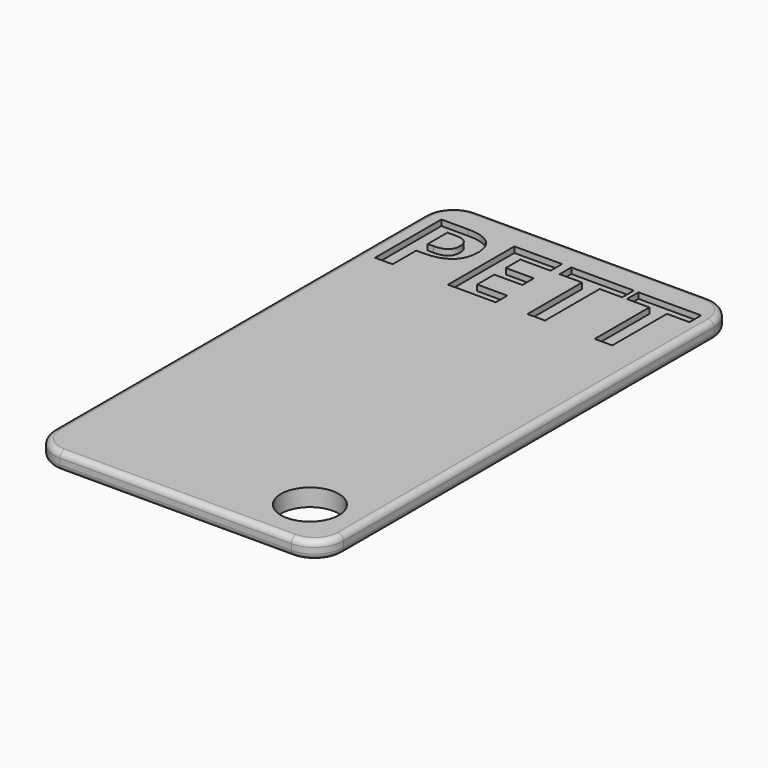
from build123d import *

# Parameters (mm, degrees)
F0_W         = 90
F0_H         = 50
F1_DEPTH     = 3
F2_R         = 1
F3_T1_DEPTH  = 3
F3_T4_ANGLE  = 90
F3_T6_ANGLE  = 90
F3_T8_ANGLE  = 90
F3_T10_ANGLE = 90
F3_T12_ANGLE = 90
F3_T14_ANGLE = 90
F3_T16_ANGLE = 90
F3_T18_ANGLE = 90
F5_ANGLE     = 90
F6_TEXT_SIZE = 20.075807084
F7_DEPTH     = 1
F8_R         = 5
F9_DEPTH     = 3


# Not quite as in the source:
# - a fillet or chamfer that OpenCascade refuses, or shapes differently, is made with other operations: its cross-section is extruded or revolved along the edge and cut away or added
# - Text() gives the source's letters only with a copy of the font that has no kerning and outlines rounded to 1/6400 em; it was checked with that copy


with BuildPart() as f1:
    # F0 (on Top) → F1 (new body)
    with BuildSketch(Plane.XY):
        Rectangle(F0_W, F0_H)
    extrude(amount=F1_DEPTH)

    # F2
    f2_edges = [f1.edges().sort_by_distance(p)[0] for p in [
        (0, 25, 3),
        (-45, 0, 3),
        (0, -25, 3),
        (45, 0, 3),
        (0, 25, 0),
        (-45, 0, 0),
        (0, -25, 0),
        (45, 0, 0),
    ]]
    fillet(f2_edges, radius=F2_R)

    # F3: fillet of radius 5 on 4 edges, made by hand

    # F3_s2 → F3_t1 (cut)
    with BuildSketch(Plane.XY):
        with BuildLine():
            ThreePointArc((45, -20), (43.5355339059, -23.5355339059), (40, -25))
            Line((40, -25), (45, -25))
            Line((45, -25), (45, -20))
        make_face()
        with BuildLine():
            ThreePointArc((40, 25), (43.5355339059, 23.5355339059), (45, 20))
            Line((45, 20), (45, 25))
            Line((45, 25), (40, 25))
        make_face()
        with BuildLine():
            ThreePointArc((-40, 25), (-43.5355339059, 23.5355339059), (-45, 20))
            Line((-45, 20), (-45, 25))
            Line((-45, 25), (-40, 25))
        make_face()
        with BuildLine():
            ThreePointArc((-45, -20), (-43.5355339059, -23.5355339059), (-40, -25))
            Line((-40, -25), (-45, -25))
            Line((-45, -25), (-45, -20))
        make_face()
    extrude(amount=F3_T1_DEPTH, mode=Mode.SUBTRACT)

    # F3_s3 → F3_t4 (revolve, cut)
    with BuildSketch(Plane.YZ.offset(-40)):
        with BuildLine():
            ThreePointArc((-24, 0), (-24.7071067812, 0.2928932188), (-25, 1))
            Line((-25, 1), (-25, 0))
            Line((-25, 0), (-24, 0))
        make_face()
    revolve(axis=Axis((-40, -20, 0), (0, 0, -1)), revolution_arc=F3_T4_ANGLE, mode=Mode.SUBTRACT)

    # F3_s5 → F3_t6 (revolve, cut)
    with BuildSketch(Plane.XZ.offset(20)):
        with BuildLine():
            ThreePointArc((-44, 3), (-44.7071067812, 2.7071067812), (-45, 2))
            Line((-45, 2), (-45, 3))
            Line((-45, 3), (-44, 3))
        make_face()
    revolve(axis=Axis((-40, -20, 3), (0, 0, 1)), revolution_arc=F3_T6_ANGLE, mode=Mode.SUBTRACT)

    # F3_s7 → F3_t8 (revolve, cut)
    with BuildSketch(Plane.XZ.offset(-20)):
        with BuildLine():
            ThreePointArc((-44, 0), (-44.7071067812, 0.2928932188), (-45, 1))
            Line((-45, 1), (-45, 0))
            Line((-45, 0), (-44, 0))
        make_face()
    revolve(axis=Axis((-40, 20, 0), (0, 0, -1)), revolution_arc=F3_T8_ANGLE, mode=Mode.SUBTRACT)

    # F3_s9 → F3_t10 (revolve, cut)
    with BuildSketch(Plane.YZ.offset(-40)):
        with BuildLine():
            ThreePointArc((24, 3), (24.7071067812, 2.7071067812), (25, 2))
            Line((25, 2), (25, 3))
            Line((25, 3), (24, 3))
        make_face()
    revolve(axis=Axis((-40, 20, 3), (0, 0, 1)), revolution_arc=F3_T10_ANGLE, mode=Mode.SUBTRACT)

    # F3_s11 → F3_t12 (revolve, cut)
    with BuildSketch(Plane.YZ.offset(40)):
        with BuildLine():
            ThreePointArc((24, 0), (24.7071067812, 0.2928932188), (25, 1))
            Line((25, 1), (25, 0))
            Line((25, 0), (24, 0))
        make_face()
    revolve(axis=Axis((40, 20, 0), (0, 0, -1)), revolution_arc=F3_T12_ANGLE, mode=Mode.SUBTRACT)

    # F3_s13 → F3_t14 (revolve, cut)
    with BuildSketch(Plane.XZ.offset(-20)):
        with BuildLine():
            ThreePointArc((44, 3), (44.7071067812, 2.7071067812), (45, 2))
            Line((45, 2), (45, 3))
            Line((45, 3), (44, 3))
        make_face()
    revolve(axis=Axis((40, 20, 3), (0, 0, 1)), revolution_arc=F3_T14_ANGLE, mode=Mode.SUBTRACT)

    # F3_s15 → F3_t16 (revolve, cut)
    with BuildSketch(Plane.XZ.offset(20)):
        with BuildLine():
            ThreePointArc((44, 0), (44.7071067812, 0.2928932188), (45, 1))
            Line((45, 1), (45, 0))
            Line((45, 0), (44, 0))
        make_face()
    revolve(axis=Axis((40, -20, 0), (0, 0, -1)), revolution_arc=F3_T16_ANGLE, mode=Mode.SUBTRACT)

    # F3_s17 → F3_t18 (revolve, cut)
    with BuildSketch(Plane.YZ.offset(40)):
        with BuildLine():
            ThreePointArc((-24, 3), (-24.7071067812, 2.7071067812), (-25, 2))
            Line((-25, 2), (-25, 3))
            Line((-25, 3), (-24, 3))
        make_face()
    revolve(axis=Axis((40, -20, 3), (0, 0, 1)), revolution_arc=F3_T18_ANGLE, mode=Mode.SUBTRACT)


with BuildPart() as f1_1:
    # F5: moved
    add(f1.part.rotate(Axis((0, 0, 16.4477843791), (0, 0, 1)), F5_ANGLE))

    # F6 (on face) → F7 (cut)
    with BuildSketch(Plane.XY.offset(3)):
        with Locations((-24, 25.80512679)):
            Text('PETT', F6_TEXT_SIZE, font='Open Sans', font_style=FontStyle.BOLD, text_align=(TextAlign.LEFT, TextAlign.BOTTOM))
    extrude(amount=-F7_DEPTH, mode=Mode.SUBTRACT)

    # F8 (on face) → F9 (cut)
    with BuildSketch(Plane.XY.offset(3)):
        with Locations((16, -36)):
            Circle(F8_R)
    extrude(amount=-F9_DEPTH, mode=Mode.SUBTRACT)


solid = f1_1.part
